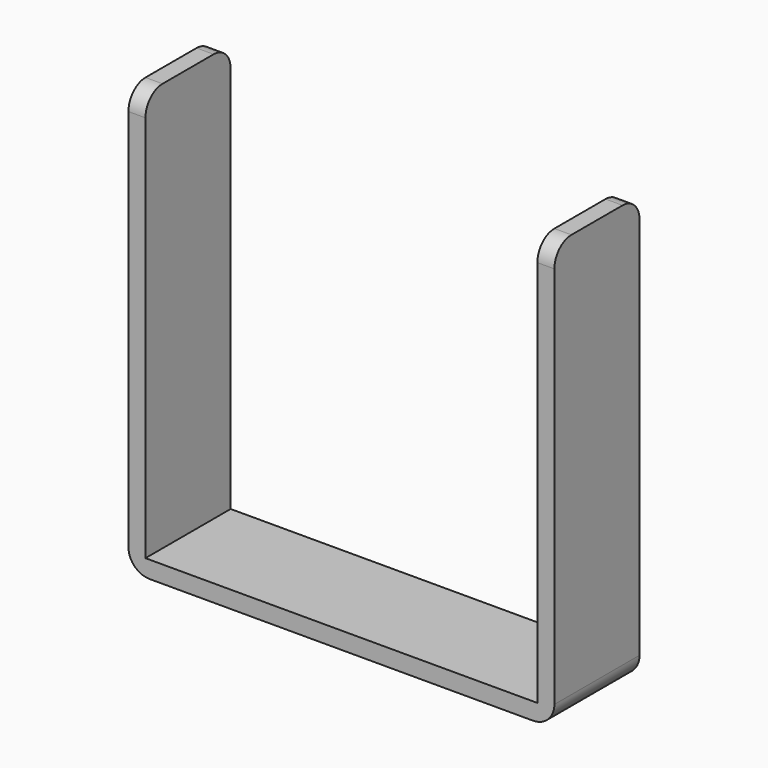
from build123d import *

# Parameters (mm, degrees)
F1_DEPTH = 12.5
F2_R     = 5


# Not quite as in the source:
# - a feature names something its author has since deleted; it is built from what else it names


with BuildPart() as f1:
    # F0 (on Front) → F1 (new body, symmetric)
    with BuildSketch(Plane.XZ):
        Polygon((-49.1098842621, 66.8063223362), (-53.1098842621, 66.8063223362), (-53.1098842621, -33.1936776638), (46.8901157379, -33.1936776638), (46.8901157379, 66.8063223362), (42.8901157379, 66.8063223362), (42.8901157379, -29.1936776638), (-49.1098842621, -29.1936776638), align=None)
    extrude(amount=F1_DEPTH, both=True)

    # F2
    f2_edges = [f1.edges().sort_by_distance(p)[0] for p in [
        (-51.109884, -12.5, 66.806322),
        (-51.109884, 12.5, 66.806322),
        (44.890116, -12.5, 66.806322),
        (44.890116, 12.5, 66.806322),
        (46.890116, 0, -33.193678),
        (-53.109884, 0, -33.193678),
    ]]
    fillet(f2_edges, radius=F2_R)


solid = f1.part
